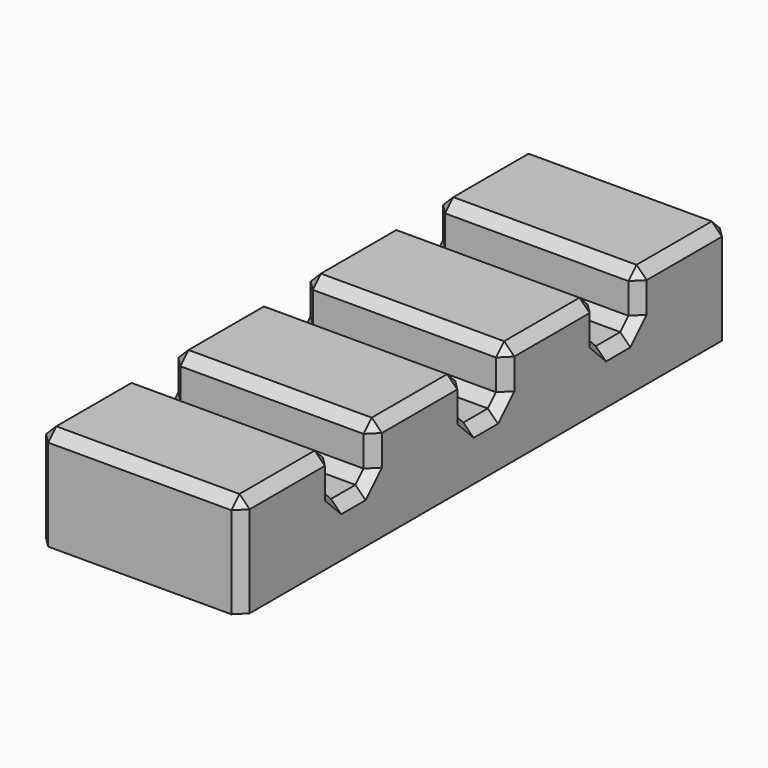
from build123d import *

# Parameters (mm, degrees)
F0_W         = 25.4
F0_H         = 76.2
F1_DEPTH     = 12.7
F2_W         = 6.35
F2_H         = 6.35
F2_H_2       = 12.7
F3_DEPTH     = 25.401
F4_SIZE      = 1.27
F5_T         = 2.54
F5_T3_DEPTH  = 6.8760512242
F5_T5_DEPTH  = 6.8760512242
F5_T7_DEPTH  = 6.8760512242
F5_T9_DEPTH  = 6.8760512242
F5_T11_DEPTH = 6.8760512242
F5_T13_DEPTH = 6.8760512242
F5_T15_DEPTH = 6.8760512242
F5_T17_DEPTH = 27.94
F5_T19_DEPTH = 6.8760512242
F5_T21_DEPTH = 6.8760512242
F5_T23_DEPTH = 6.8760512242
F5_T25_DEPTH = 6.8760512242
F5_T27_DEPTH = 6.8760512242
F5_T29_DEPTH = 6.8760512242
F5_T31_DEPTH = 6.8760512242


# Not quite as in the source:
# - a shell that OpenCascade refuses in one call is made with other operations: the cavity is built on its own and cut out


with BuildPart() as f1:
    # F0 (on Top) → F1 (new body)
    with BuildSketch(Plane.XY):
        Rectangle(F0_W, F0_H)
    extrude(amount=F1_DEPTH)

    # F2 (on face) → F3 (cut, through all)
    with BuildSketch(Plane(origin=(-12.7, 0, 0), x_dir=(0, -1, 0), z_dir=(-1, 0, 0))):
        with Locations((-20.6502, 9.525)):
            Rectangle(F2_W, F2_H)
        with Locations((-20.6502, 15.875)):
            Rectangle(F2_W, F2_H)
        with Locations((0, 15.875)):
            Rectangle(F2_W, F2_H)
        with Locations((0, 9.525)):
            Rectangle(F2_W, F2_H)
        with Locations((20.6502, 9.525)):
            Rectangle(F2_W, F2_H)
        with Locations((20.6502, 15.875)):
            Rectangle(F2_W, F2_H)
        with Locations((0, 12.7)):
            Rectangle(F2_W, F2_H_2)
        with Locations((20.6502, 12.7)):
            Rectangle(F2_W, F2_H_2)
        with Locations((-20.6502, 12.7)):
            Rectangle(F2_W, F2_H_2)
    extrude(amount=-F3_DEPTH, mode=Mode.SUBTRACT)

    # F4
    f4_edges = [f1.edges().sort_by_distance(p)[0] for p in [
        (0, -3.175, 12.7),
        (12.7, -10.3251, 12.7),
        (0, -17.4752, 12.7),
        (-12.7, -10.3251, 12.7),
        (0, 38.1, 12.7),
        (12.7, 30.9626, 12.7),
        (0, 23.8252, 12.7),
        (-12.7, 30.9626, 12.7),
        (-12.7, 0, 6.35),
        (0, -3.175, 6.35),
        (12.7, 0, 6.35),
        (0, 3.175, 6.35),
        (-12.7, -20.6502, 6.35),
        (0, -23.8252, 6.35),
        (12.7, -20.6502, 6.35),
        (0, -17.4752, 6.35),
        (-12.7, 20.6502, 6.35),
        (0, 17.4752, 6.35),
        (12.7, 20.6502, 6.35),
        (0, 23.8252, 6.35),
        (0, 17.4752, 12.7),
        (12.7, 10.3251, 12.7),
        (0, 3.175, 12.7),
        (-12.7, 10.3251, 12.7),
        (0, -23.8252, 12.7),
        (12.7, -30.9626, 12.7),
        (0, -38.1, 12.7),
        (-12.7, -30.9626, 12.7),
        (-12.7, 38.1, 6.35),
        (12.7, 38.1, 6.35),
        (-12.7, -38.1, 6.35),
        (12.7, -38.1, 6.35),
        (-12.7, -23.8252, 9.525),
        (-12.7, -17.4752, 9.525),
        (-12.7, -3.175, 9.525),
        (-12.7, 3.175, 9.525),
        (-12.7, 17.4752, 9.525),
        (-12.7, 23.8252, 9.525),
        (12.7, -23.8252, 9.525),
        (12.7, -17.4752, 9.525),
        (12.7, -3.175, 9.525),
        (12.7, 3.175, 9.525),
        (12.7, 17.4752, 9.525),
        (12.7, 23.8252, 9.525),
    ]]
    chamfer(f4_edges, length=F4_SIZE)

    # F5: shell of thickness 2.54, made by hand


with BuildPart() as f5_core1:
    # F5_t2: copy of F1
    add(f1.part)

    # the walls: a layer under each face that stays
    f5_faces = [f5_core1.faces().sort_by_distance(p)[0] for p in [
        (-12.7, 24.5533333333, 5.715),
        (-12.065, 37.465, 5.715),
        (-12.065, -37.465, 5.715),
        (-12.065, 30.9626, 12.065),
        (-12.065, -30.9626, 12.065),
        (-12.065, 24.4602, 9.525),
        (-12.065, -24.4602, 9.525),
        (-12.065, 23.5077, 6.6675),
        (-12.065, -23.5077, 6.6675),
        (-12.065, 20.6502, 5.715),
        (-12.065, -20.6502, 5.715),
        (-12.065, 17.7927, 6.6675),
        (-12.065, -17.7927, 6.6675),
        (-12.065, 16.8402, 9.525),
        (-12.065, -16.8402, 9.525),
        (-12.065, 10.3251, 12.065),
        (-12.065, -10.3251, 12.065),
        (-12.065, 3.81, 9.525),
        (-12.065, -3.81, 9.525),
        (-12.065, 2.8575, 6.6675),
        (-12.065, -2.8575, 6.6675),
        (-12.065, 0, 5.715),
        (0, 38.1, 5.715),
        (0, -38.1, 5.715),
        (12.065, 37.465, 5.715),
        (12.065, -37.465, 5.715),
        (12.7, -24.5533333333, 5.715),
        (-12.065, 37.1475, 11.7475),
        (-12.065, -37.1475, 11.7475),
        (0, 30.9626, 12.7),
        (-12.065, 24.7777, 11.7475),
        (-12.065, -24.7777, 11.7475),
        (0, -30.9626, 12.7),
        (0, 23.8252, 9.525),
        (0, -23.8252, 9.525),
        (0, 23.1902, 6.985),
        (0, -23.1902, 6.985),
        (0, 20.6502, 6.35),
        (0, -20.6502, 6.35),
        (0, 18.1102, 6.985),
        (0, -18.1102, 6.985),
        (0, 17.4752, 9.525),
        (-12.065, 16.5227, 11.7475),
        (-12.065, -16.5227, 11.7475),
        (0, -17.4752, 9.525),
        (0, 10.3251, 12.7),
        (-12.065, 4.1275, 11.7475),
        (-12.065, -4.1275, 11.7475),
        (0, -10.3251, 12.7),
        (0, 3.175, 9.525),
        (0, -3.175, 9.525),
        (0, 2.54, 6.985),
        (0, -2.54, 6.985),
        (0, 0, 6.35),
        (0, 37.465, 12.065),
        (0, -37.465, 12.065),
        (12.065, 37.1475, 11.7475),
        (11.7475, -37.465, 11.7475),
        (12.065, -30.9626, 12.065),
        (12.065, 30.9626, 12.065),
        (12.065, -24.4602, 9.525),
        (12.065, 24.4602, 9.525),
        (12.065, -23.5077, 6.6675),
        (12.065, 23.5077, 6.6675),
        (12.065, -20.6502, 5.715),
        (12.065, 20.6502, 5.715),
        (12.065, -17.7927, 6.6675),
        (12.065, 17.7927, 6.6675),
        (12.065, -16.8402, 9.525),
        (12.065, 16.8402, 9.525),
        (12.065, -10.3251, 12.065),
        (12.065, 10.3251, 12.065),
        (12.065, -3.81, 9.525),
        (12.065, 3.81, 9.525),
        (12.065, -2.8575, 6.6675),
        (12.065, 2.8575, 6.6675),
        (12.065, 0, 5.715),
        (0, 24.4602, 12.065),
        (0, -24.4602, 12.065),
        (0, 16.8402, 12.065),
        (0, -16.8402, 12.065),
        (0, 3.81, 12.065),
        (0, -3.81, 12.065),
        (12.065, -24.7777, 11.7475),
        (11.7475, 24.4602, 11.7475),
        (11.7475, -16.8402, 11.7475),
        (12.065, 16.5227, 11.7475),
        (12.065, -4.1275, 11.7475),
        (11.7475, 3.81, 11.7475),
    ]]
    thicken(f5_faces, amount=-F5_T, mode=Mode.SUBTRACT)

    # F5_s4 → F5_t3 (cut)
    with BuildSketch(Plane(origin=(-20.6936512242, 20.6936512242, 0), x_dir=(0, 0, 1), z_dir=(0.7071067812, -0.7071067812, 0))):
        Polygon((7.6346646968, -8.718590961), (7.62, -11.3047299742), (6.8126933972, -11.3047299742), (6.1535303163, -10.8386312897), align=None)
    extrude(amount=F5_T3_DEPTH, mode=Mode.SUBTRACT)

    # F5_s6 → F5_t5 (cut)
    with BuildSketch(Plane(origin=(-20.6936512242, -20.6936512242, 0), x_dir=(0, 0, 1), z_dir=(0.7071067812, 0.7071067812, 0))):
        Polygon((7.6346646968, 8.718590961), (7.62, 11.3047299742), (6.8126933972, 11.3047299742), (6.1535303163, 10.8386312897), align=None)
    extrude(amount=F5_T5_DEPTH, mode=Mode.SUBTRACT)

    # F5_s8 → F5_t7 (cut)
    with BuildSketch(Plane(origin=(-5.6060512242, 0, -5.6060512242), x_dir=(0, 1, 0), z_dir=(0.7071067812, 0, 0.7071067812))):
        Polygon((22.5405353032, 12.6184975827), (24.0216696837, 10.4984572539), (23.3625066028, 10.0323585695), (22.5552, 10.0323585695), align=None)
        Polygon((-22.5405353032, 12.6184975827), (-24.0216696837, 10.4984572539), (-23.3625066028, 10.0323585695), (-22.5552, 10.0323585695), align=None)
        Polygon((18.7598646968, 12.6184975827), (18.7452, 10.0323585695), (17.9378933972, 10.0323585695), (17.2787303163, 10.4984572539), align=None)
        Polygon((-18.7598646968, 12.6184975827), (-18.7452, 10.0323585695), (-17.9378933972, 10.0323585695), (-17.2787303163, 10.4984572539), align=None)
        Polygon((1.8903353032, 12.6184975827), (3.3714696837, 10.4984572539), (2.7123066028, 10.0323585695), (1.905, 10.0323585695), align=None)
        Polygon((-1.8903353032, 12.6184975827), (-3.3714696837, 10.4984572539), (-2.7123066028, 10.0323585695), (-1.905, 10.0323585695), align=None)
    extrude(amount=F5_T7_DEPTH, mode=Mode.SUBTRACT)

    # F5_s10 → F5_t9 (cut)
    with BuildSketch(Plane(origin=(-0.0434512242, -0.0434512242, 0), x_dir=(0, 0, 1), z_dir=(0.7071067812, 0.7071067812, 0))):
        Polygon((7.6346646968, -20.4852019447), (6.1535303163, -18.365161616), (6.8126933972, -17.8990629316), (7.62, -17.8990629316), align=None)
    extrude(amount=F5_T9_DEPTH, mode=Mode.SUBTRACT)

    # F5_s12 → F5_t11 (cut)
    with BuildSketch(Plane(origin=(-0.0434512242, 0.0434512242, 0), x_dir=(0, 0, 1), z_dir=(0.7071067812, -0.7071067812, 0))):
        Polygon((7.6346646968, 20.4852019447), (6.1535303163, 18.365161616), (6.8126933972, 17.8990629316), (7.62, 17.8990629316), align=None)
    extrude(amount=F5_T11_DEPTH, mode=Mode.SUBTRACT)

    # F5_s14 → F5_t13 (cut)
    with BuildSketch(Plane(origin=(-10.3685512242, 10.3685512242, 0), x_dir=(0, 0, 1), z_dir=(0.7071067812, -0.7071067812, 0))):
        Polygon((7.6346646968, 5.8833054919), (7.62, 3.2971664787), (6.8126933972, 3.2971664787), (6.1535303163, 3.7632651631), align=None)
    extrude(amount=F5_T13_DEPTH, mode=Mode.SUBTRACT)

    # F5_s16 → F5_t15 (cut)
    with BuildSketch(Plane(origin=(-10.3685512242, -10.3685512242, 0), x_dir=(0, 0, 1), z_dir=(0.7071067812, 0.7071067812, 0))):
        Polygon((7.6346646968, -5.8833054919), (7.62, -3.2971664787), (6.8126933972, -3.2971664787), (6.1535303163, -3.7632651631), align=None)
    extrude(amount=F5_T15_DEPTH, mode=Mode.SUBTRACT)

    # F5_s18 → F5_t17 (cut)
    with BuildSketch(Plane.YZ.offset(-13.97)):
        Polygon((23.7818394878, 7.6379605122), (26.3652, 7.62), (26.3652, 6.5678975516), (25.6212512242, 5.8239487758), align=None)
        Polygon((-23.7818394878, 7.6379605122), (-26.3652, 7.62), (-26.3652, 6.5678975516), (-25.6212512242, 5.8239487758), align=None)
        Polygon((22.5372394878, 6.3933605122), (24.3512512242, 4.5539487758), (23.6073024484, 3.81), (22.5552, 3.81), align=None)
        Polygon((-22.5372394878, 6.3933605122), (-24.3512512242, 4.5539487758), (-23.6073024484, 3.81), (-22.5552, 3.81), align=None)
        Polygon((18.7631605122, 6.3933605122), (18.7452, 3.81), (17.6930975516, 3.81), (16.9491487758, 4.5539487758), align=None)
        Polygon((-18.7631605122, 6.3933605122), (-18.7452, 3.81), (-17.6930975516, 3.81), (-16.9491487758, 4.5539487758), align=None)
        Polygon((17.5185605122, 7.6379605122), (15.6791487758, 5.8239487758), (14.9352, 6.5678975516), (14.9352, 7.62), align=None)
        Polygon((-17.5185605122, 7.6379605122), (-15.6791487758, 5.8239487758), (-14.9352, 6.5678975516), (-14.9352, 7.62), align=None)
        Polygon((3.1316394878, 7.6379605122), (5.715, 7.62), (5.715, 6.5678975516), (4.9710512242, 5.8239487758), align=None)
        Polygon((-3.1316394878, 7.6379605122), (-5.715, 7.62), (-5.715, 6.5678975516), (-4.9710512242, 5.8239487758), align=None)
        Polygon((1.8870394878, 6.3933605122), (3.7010512242, 4.5539487758), (2.9571024484, 3.81), (1.905, 3.81), align=None)
        Polygon((-1.8870394878, 6.3933605122), (-3.7010512242, 4.5539487758), (-2.9571024484, 3.81), (-1.905, 3.81), align=None)
    extrude(amount=F5_T17_DEPTH, mode=Mode.SUBTRACT)

    # F5_s20 → F5_t19 (cut)
    with BuildSketch(Plane(origin=(20.6936512242, -20.6936512242, 0), x_dir=(0, 0, 1), z_dir=(-0.7071067812, 0.7071067812, 0))):
        Polygon((7.6346646968, -8.718590961), (7.62, -11.3047299742), (6.8126933972, -11.3047299742), (6.1535303163, -10.8386312897), align=None)
    extrude(amount=F5_T19_DEPTH, mode=Mode.SUBTRACT)

    # F5_s22 → F5_t21 (cut)
    with BuildSketch(Plane(origin=(20.6936512242, 20.6936512242, 0), x_dir=(0, 0, 1), z_dir=(-0.7071067812, -0.7071067812, 0))):
        Polygon((7.6346646968, 8.718590961), (7.62, 11.3047299742), (6.8126933972, 11.3047299742), (6.1535303163, 10.8386312897), align=None)
    extrude(amount=F5_T21_DEPTH, mode=Mode.SUBTRACT)

    # F5_s24 → F5_t23 (cut)
    with BuildSketch(Plane(origin=(5.6060512242, 0, -5.6060512242), x_dir=(0, 1, 0), z_dir=(-0.7071067812, 0, 0.7071067812))):
        Polygon((-22.5405353032, -12.6184975827), (-24.0216696837, -10.4984572539), (-23.3625066028, -10.0323585695), (-22.5552, -10.0323585695), align=None)
        Polygon((22.5405353032, -12.6184975827), (24.0216696837, -10.4984572539), (23.3625066028, -10.0323585695), (22.5552, -10.0323585695), align=None)
        Polygon((-18.7598646968, -12.6184975827), (-18.7452, -10.0323585695), (-17.9378933972, -10.0323585695), (-17.2787303163, -10.4984572539), align=None)
        Polygon((18.7598646968, -12.6184975827), (18.7452, -10.0323585695), (17.9378933972, -10.0323585695), (17.2787303163, -10.4984572539), align=None)
        Polygon((-1.8903353032, -12.6184975827), (-3.3714696837, -10.4984572539), (-2.7123066028, -10.0323585695), (-1.905, -10.0323585695), align=None)
        Polygon((1.8903353032, -12.6184975827), (3.3714696837, -10.4984572539), (2.7123066028, -10.0323585695), (1.905, -10.0323585695), align=None)
    extrude(amount=F5_T23_DEPTH, mode=Mode.SUBTRACT)

    # F5_s26 → F5_t25 (cut)
    with BuildSketch(Plane(origin=(0.0434512242, 0.0434512242, 0), x_dir=(0, 0, 1), z_dir=(-0.7071067812, -0.7071067812, 0))):
        Polygon((7.6346646968, -20.4852019447), (6.1535303163, -18.365161616), (6.8126933972, -17.8990629316), (7.62, -17.8990629316), align=None)
    extrude(amount=F5_T25_DEPTH, mode=Mode.SUBTRACT)

    # F5_s28 → F5_t27 (cut)
    with BuildSketch(Plane(origin=(0.0434512242, -0.0434512242, 0), x_dir=(0, 0, 1), z_dir=(-0.7071067812, 0.7071067812, 0))):
        Polygon((7.6346646968, 20.4852019447), (6.1535303163, 18.365161616), (6.8126933972, 17.8990629316), (7.62, 17.8990629316), align=None)
    extrude(amount=F5_T27_DEPTH, mode=Mode.SUBTRACT)

    # F5_s30 → F5_t29 (cut)
    with BuildSketch(Plane(origin=(10.3685512242, -10.3685512242, 0), x_dir=(0, 0, 1), z_dir=(-0.7071067812, 0.7071067812, 0))):
        Polygon((7.6346646968, 5.8833054919), (7.62, 3.2971664787), (6.8126933972, 3.2971664787), (6.1535303163, 3.7632651631), align=None)
    extrude(amount=F5_T29_DEPTH, mode=Mode.SUBTRACT)

    # F5_s32 → F5_t31 (cut)
    with BuildSketch(Plane(origin=(10.3685512242, 10.3685512242, 0), x_dir=(0, 0, 1), z_dir=(-0.7071067812, -0.7071067812, 0))):
        Polygon((7.6346646968, -5.8833054919), (7.62, -3.2971664787), (6.8126933972, -3.2971664787), (6.1535303163, -3.7632651631), align=None)
    extrude(amount=F5_T31_DEPTH, mode=Mode.SUBTRACT)


with BuildPart() as f1_1:
    add(f1.part)

    # what is left inside the walls is the cavity
    f5_cavity = [f5_core1.part.solids().sort_by_distance(p)[0] for p in [
        (0, -11.853333, 0.0254),
    ]]
    add(f5_cavity, mode=Mode.SUBTRACT)


solid = f1_1.part
